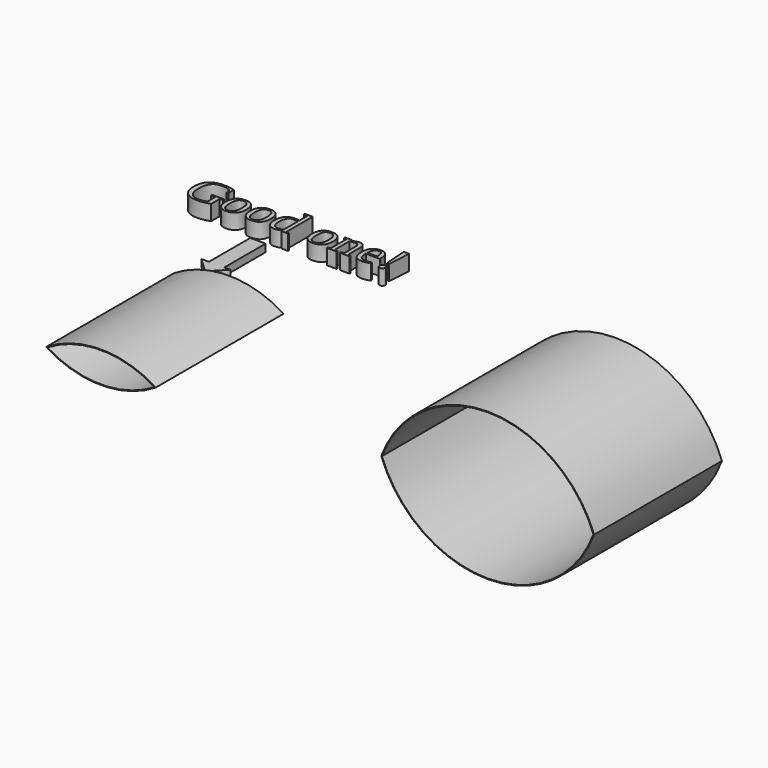
from build123d import *

# Parameters (mm, degrees)
F1_DEPTH     = 100.2538
F3_DEPTH     = 100.2792
F4_TEXT_SIZE = 31.0365524557
F5_DEPTH     = 9.6012
F6_W         = 9.6480101347
F6_H         = 32.4361100793
F7_DEPTH     = 4.7625


# Not quite as in the source:
# - Text() gives the source's letters only with a copy of the font that has no kerning and outlines rounded to 1/6400 em; it was checked with that copy


with BuildPart() as f1:
    # F0 (on Front) → F1 (new body)
    with BuildSketch(Plane.XZ):
        with BuildLine():
            ThreePointArc((94.2913672312, 8.1395031661), (161.1146330833, -38.2036201775), (227.9378989355, 8.1395031661))
            ThreePointArc((227.9378989355, 8.1395031661), (161.1146330833, 54.4826265097), (94.2913672312, 8.1395031661))
        make_face()
        with BuildLine():
            ThreePointArc((94.7254631983, 8.1395031661), (161.1146330833, 54.0762265097), (227.5038029684, 8.1395031661))
            ThreePointArc((227.5038029684, 8.1395031661), (161.1146330833, -37.7972201775), (94.7254631983, 8.1395031661))
        make_face(mode=Mode.SUBTRACT)
    extrude(amount=F1_DEPTH)


with BuildPart() as f3:
    # F2 (on Front) → F3 (new body)
    with BuildSketch(Plane.XZ):
        with BuildLine():
            ThreePointArc((-116.042025411, 0), (-81.5899540319, -9.8909556365), (-47.1378826528, 0))
            ThreePointArc((-47.1378826528, 0), (-81.5899540319, 9.8909556365), (-116.042025411, 0))
        make_face()
        with BuildLine():
            ThreePointArc((-115.2696429234, 0), (-81.5899540319, 9.4845556365), (-47.9102651404, 0))
            ThreePointArc((-47.9102651404, 0), (-81.5899540319, -9.4845556365), (-115.2696429234, 0))
        make_face(mode=Mode.SUBTRACT)
    extrude(amount=F3_DEPTH)


with BuildPart() as f5:
    # F4 (on Top) → F5 (new body)
    with BuildSketch(Plane.XY):
        with Locations((-155.7046622038, 53.3812195063)):
            Text('Good one!', F4_TEXT_SIZE, font='Tinos', text_align=(TextAlign.LEFT, TextAlign.BOTTOM))
    extrude(amount=F5_DEPTH)


with BuildPart() as f7:
    # F6 (on Top) → F7 (new body)
    with BuildSketch(Plane.XY):
        with Locations((-99.6469631791, 29.2668454349)):
            Rectangle(F6_W, F6_H)
        Polygon((-94.8229581118, 13.0487903953), (-104.4709682465, 13.0487903953), (-109.1885566711, 13.0487903953), (-99.6469631791, 3.9382465184), (-90.9479958838, 13.0487903953), align=None)
    extrude(amount=F7_DEPTH)


solid = Compound([f1.part, f3.part, f5.part, f7.part])
